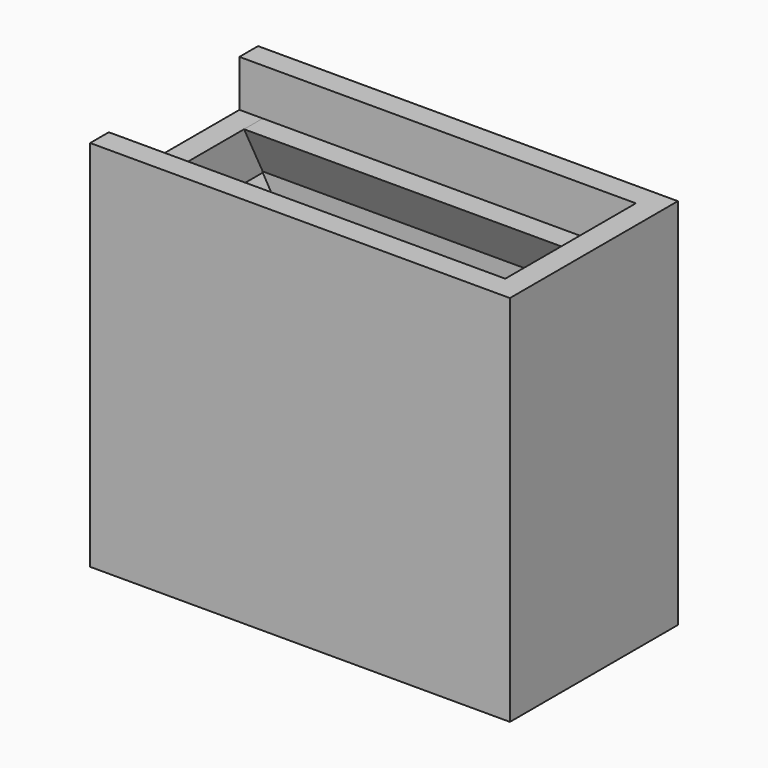
from build123d import *

# Parameters (mm, degrees)
F0_W      = 18
F0_H      = 9
F1_DEPTH  = 14
F2_W      = 16
F2_H      = 7
F3_DEPTH  = 7
F4_W      = 4
F4_H      = 4
F5_DEPTH  = 6
F4_W_2    = 2.5
F4_H_2    = 7
F6_DEPTH  = 9
F8_DEPTH  = 2
F10_DEPTH = 7
F12_DEPTH = 16
F13_W     = 3
F13_H     = 5.4984997745
F14_DEPTH = 10


with BuildPart() as f1:
    # F0 (on Top) → F1 (new body)
    with BuildSketch(Plane.XY):
        Rectangle(F0_W, F0_H)
    extrude(amount=F1_DEPTH)

    # F2 (on face) → F3 (cut)
    with BuildSketch(Plane.XY.offset(14)):
        Rectangle(F2_W, F2_H)
    extrude(amount=-F3_DEPTH, mode=Mode.SUBTRACT)

    # F4 (on face) → F5 (cut)
    with BuildSketch(Plane(origin=(0, 0, 0), x_dir=(1, 0, 0), z_dir=(0, 0, -1))):
        with Locations((2.1, 0)):
            Rectangle(F4_W, F4_H)
    extrude(amount=-F5_DEPTH, mode=Mode.SUBTRACT)

    # F4 (on face) → F6 (cut)
    with BuildSketch(Plane(origin=(0, 0, 0), x_dir=(1, 0, 0), z_dir=(0, 0, -1))):
        with Locations((-6.75, 0)):
            Rectangle(F4_W_2, F4_H_2)
    extrude(amount=-F6_DEPTH, mode=Mode.SUBTRACT)

    # F7 (on face) → F8 (join)
    with BuildSketch(Plane.XY.offset(14)):
        Polygon((9, 4.5), (-9, 4.5), (-9, 3.5), (8, 3.5), (8, -3.5), (-9, -3.5), (-9, -4.5), (9, -4.5), align=None)
    extrude(amount=F8_DEPTH)


with BuildPart() as f10:
    # F9 (on face) → F10 (new body)
    with BuildSketch(Plane(origin=(0, -3.5, 0), x_dir=(-1, 0, 0), z_dir=(0, 1, 0))):
        Polygon((-7, 14), (-8, 14), (-8, 12), align=None)
    extrude(amount=F10_DEPTH)

    # F11 (on face) → F12 (join)
    with BuildSketch(Plane(origin=(8, 0, 0), x_dir=(0, -1, 0), z_dir=(-1, 0, 0))):
        Polygon((3.5, 12), (3.5, 14), (2.5, 14), align=None)
        Polygon((-3.5, 12), (-2.5, 14), (-3.5, 14), align=None)
    extrude(amount=F12_DEPTH)


with BuildPart() as f10b:
    # F9 (on face) → F10, piece 2 (new body)
    with BuildSketch(Plane(origin=(0, -3.5, 0), x_dir=(-1, 0, 0), z_dir=(0, 1, 0))):
        Polygon((-8, 11.9536653096), (-8, 7), (-5.14, 7), align=None)
    extrude(amount=F10_DEPTH)


with BuildPart() as f10c:
    # F9 (on face) → F10, piece 3 (new body)
    with BuildSketch(Plane(origin=(0, -3.5, 0), x_dir=(-1, 0, 0), z_dir=(0, 1, 0))):
        Polygon((8, 7), (8, 11.9536653096), (5.14, 7), align=None)
    extrude(amount=F10_DEPTH)

    # F13 (on face) → F14 (cut)
    with BuildSketch(Plane(origin=(-9, 0, 0), x_dir=(0, -1, 0), z_dir=(-1, 0, 0))):
        with Locations((0, 9.0919707436)):
            Rectangle(F13_W, F13_H)
    extrude(amount=-F14_DEPTH, mode=Mode.SUBTRACT)


solid = Compound([f1.part, f10.part, f10b.part, f10c.part])
